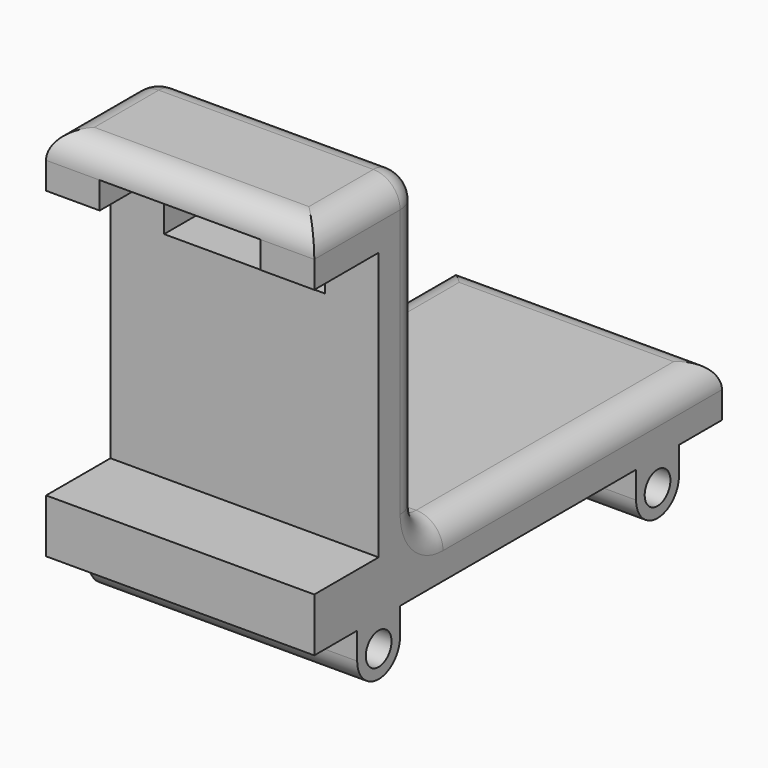
from build123d import *

# Parameters (mm, degrees)
F1_DEPTH = 50
F2_F1_R  = 5
F2_F2_R  = 5
F3_W     = 10
F3_H     = 10
F3_R     = 3
F4_DEPTH = 50
F5_R     = 4.99999
F6_W     = 30
F6_H     = 14.961473023
F7_DEPTH = 25


# Not quite as in the source:
# - a fillet or chamfer is up to 0.001 mm smaller than in the source, because OpenCascade refuses the exact size


with BuildPart() as f1:
    # F0 (on Right) → F1 (new body)
    with BuildSketch(Plane.YZ):
        Polygon((-95, 0), (0, 0), (0, 10), (-70, 10), (-70, 70), (-82.7777751063, 70), (-95, 70), (-95, 60), (-80, 60), (-80, 10), (-95, 10), align=None)
    extrude(amount=F1_DEPTH)

    # F2: fillet of radius 5 on 8 edges, made by hand

    # F2_f1
    f2_f1_edges = [f1.edges().sort_by_distance(p)[0] for p in [
        (25, -70, 10),
    ]]
    fillet(f2_f1_edges, radius=F2_F1_R)

    # F2_f2
    f2_f2_edges = [f1.edges().sort_by_distance(p)[0] for p in [
        (25, -70, 70),
        (50, -82.5, 70),
        (0, -82.5, 70),
        (25, 0, 10),
        (50, -32.5, 10),
        (0, -32.5, 10),
        (25, -95, 70),
        (0, -68.5355339059, 11.4644660941),
        (50, -68.5355339059, 11.4644660941),
    ]]
    fillet(f2_f2_edges, radius=F2_F2_R)

    # F3 (on face) → F4 (join)
    with BuildSketch(Plane.YZ.offset(50)):
        with Locations((-80, -5)):
            Rectangle(F3_W, F3_H)
        with Locations((-80, -5)):
            Circle(F3_R, mode=Mode.SUBTRACT)
        with Locations((-15, -5)):
            Rectangle(F3_W, F3_H)
        with Locations((-15, -5)):
            Circle(F3_R, mode=Mode.SUBTRACT)
    extrude(amount=-F4_DEPTH)

    # F5 (radius 5 in the source; OpenCascade refuses exactly that, so slightly less here)
    f5_edges = [f1.edges().sort_by_distance(p)[0] for p in [
        (25, -75, -10),
        (25, -85, -10),
        (25, -20, -10),
        (25, -10, -10),
    ]]
    fillet(f5_edges, radius=F5_R)

    # F6 (on face) → F7 (cut)
    with BuildSketch(Plane(origin=(0, -70, 0), x_dir=(-1, 0, 0), z_dir=(0, 1, 0))):
        with Locations((-25, 57.5192634885)):
            Rectangle(F6_W, F6_H)
    extrude(amount=-F7_DEPTH, mode=Mode.SUBTRACT)


solid = f1.part
